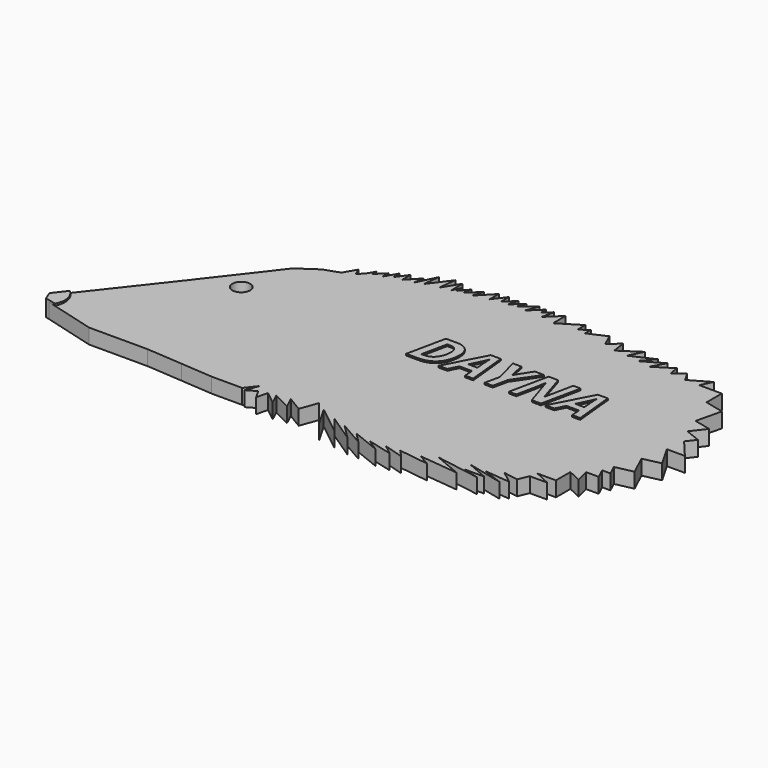
from build123d import *

# Parameters (mm, degrees)
F0_R         = 0.5378033018
F1_DEPTH     = 0.9
F2_TEXT_SIZE = 3.3063238435
F3_DEPTH     = 1
F5_DEPTH     = 1.01


# Not quite as in the source:
# - Text() gives the source's letters only with a copy of the font that has no kerning and outlines rounded to 1/6400 em; it was checked with that copy


with BuildPart() as f1:
    # F0 (on Top) → F1 (new body)
    with BuildSketch(Plane.XY):
        Polygon((-27.0037204027, 5.1291389391), (-31.1524681747, -0.163565157), (-30.9421550483, -0.6564339856), (-27.6378747076, -1.5638275072), (-24.1281446069, -1.5638275072), (-21.9538230449, -1.7179133138), (-20.0191922486, -1.8652107101), (-18.1791530636, -1.8652107101), (-17.6565442234, -1.1985001504), (-17.9531408334, -1.9743070749), (-17.3907472424, -1.6495448565), (-17.0744433999, -2.1972910035), (-16.9113259139, -1.5163020821), (-16.1478312427, -2.1147762757), (-16.4409801364, -1.4782244107), (-15.3690173699, -2.0160753835), (-15.6876724213, -1.3241387205), (-14.780279249, -1.8652107101), (-14.3968500197, -0.8131673094), (-13.0864167586, -2.4542018443), (-13.8115396517, -1.1985001504), (-12.0932376012, -2.5454112329), (-12.8187853843, -1.6203386476), (-11.1681651324, -2.7177287266), (-12.020682916, -1.8652107101), (-10.4970345274, -2.7358673979), (-11.086541228, -2.1372910123), (-9.4268526882, -2.799352631), (-10.1433303207, -2.3368163966), (-8.6197278335, -2.7334264399), (-9.2182578519, -2.2642617114), (-8.0029657111, -2.6270351373), (-8.4055373445, -2.2042002529), (-6.5982462838, -2.448795829), (-7.2912680916, -2.0547248423), (-4.9540190957, -2.299320884), (-6.5574799664, -1.6198880039), (-3.8941039238, -2.0683135372), (-4.8724873923, -1.8101290334), (-3.6630968098, -1.8101290334), (-4.9540190957, -1.2529940577), (-2.7526570484, -1.7829518765), (-3.9892247878, -1.3345261104), (-2.4316561306, -1.484446951), (-3.1603167299, -0.9132778505), (-2.2906428203, -1.0627531447), (-2.0188696217, -0.4376749566), (-0.9725430864, -0.4376749566), (-1.9101604121, 0), (-0.7958906353, 0), (-0.7958906353, 1.0842544725), (0, 0.7173608174), (-0.2115784591, 1.5355834401), (0.54776415, 1.5355834401), (0.2640244784, 2.151703852), (0.7583171951, 2.151703852), (0.4762638127, 2.7641626075), (1.5363685326, 2.9920388722), (0.9654549067, 4.2317369953), (2.0177976039, 4.4688973236), (1.2915831758, 5.7264892384), (2.3786751553, 5.7264892384), (1.4246247635, 6.8606109064), (1.8351287581, 7.3843053542), (0.9124764773, 7.7600274963), (1.5557164371, 8.5806314368), (0.54776415, 8.8206200221), (0.9111003601, 10.3466324508), (-0.2303463552, 10.6184054166), (-0.2303463552, 11.7648066953), (-1.5892117517, 11.7648066953), (-1.2599784476, 12.4465006899), (-2.4404739359, 11.7648066953), (-2.7649223339, 12.3266568407), (-3.3876749221, 11.8695907295), (-3.4910559189, 12.4540766701), (-4.5975148678, 11.7648066953), (-4.1440478526, 12.5810466707), (-5.431894213, 11.8373613805), (-4.7426242381, 12.6173244789), (-6.1211637221, 11.9824707508), (-5.7039740495, 12.816850096), (-6.9011272863, 12.0187476277), (-7.0280982181, 12.8349885345), (-7.6510727601, 12.2644306361), (-7.9894484952, 13.0163757131), (-9.0777678415, 12.5266313553), (-9.0777678415, 12.9800979048), (-9.5856515691, 12.5991860405), (-9.5856515691, 13.1977619603), (-10.8916368335, 12.3996604234), (-10.8916368335, 13.3428713307), (-11.7078768089, 12.5629082322), (-11.5446290001, 13.3065944538), (-12.0162339881, 12.8712663427), (-12.0162339881, 13.2703166455), (-12.7417817712, 12.5629082322), (-12.4334236607, 13.3247328922), (-13.2859414443, 12.6536013559), (-13.0864167586, 13.1614850834), (-13.7394089252, 12.5629082322), (-13.576160185, 13.1433457136), (-14.1747370362, 12.5810466707), (-14.1747370362, 13.1796235219), (-14.7370360792, 12.4359373003), (-14.7370360792, 13.1252072752), (-15.6258307397, 12.2001348063), (-15.4081676155, 12.8531269729), (-16.1325391382, 12.182071805), (-16.0235837102, 12.6784220338), (-16.4715088904, 12.1578592807), (-16.4715088904, 12.5210424885), (-16.7136322707, 12.0125859976), (-16.7136322707, 12.8842266276), (-17.3310432583, 11.8794189766), (-17.2099824995, 12.9447570071), (-18.1179400533, 11.7220394313), (-18.008986488, 12.7026345581), (-18.5900796205, 11.5041295066), (-18.4811241925, 12.1578592807), (-19.1832799464, 11.4193866029), (-19.1832799464, 12.0610101148), (-19.6796301752, 11.3709615543), (-19.6796301752, 11.8431001902), (-20.1033446938, 11.1167337745), (-20.1033446938, 11.5404473618), (-20.6481199712, 10.9956720844), (-20.6481199712, 11.3104311749), (-20.9265593439, 10.8503988013), (-21.2534256279, 10.5114271864), (-21.4350167662, 10.9472479671), (-21.8708366156, 10.208774358), (-22.8030085564, 9.8819099367), (-23.9167697728, 9.1192247346), align=None)
        with Locations((-24.6249865741, 6.1201211065)):
            Circle(F0_R, mode=Mode.SUBTRACT)
    extrude(amount=F1_DEPTH)

    # F2 (on Top) → F3 (join)
    with BuildSketch(Plane.XY):
        with Locations((-14.3002690747, 5.5137877353)):
            Text('DAYNA', F2_TEXT_SIZE, font='Open Sans', font_style=FontStyle.BOLDITALIC, text_align=(TextAlign.LEFT, TextAlign.BOTTOM))
    extrude(amount=F3_DEPTH)

    # F4 (on Top) → F5 (join)
    with BuildSketch(Plane.XY):
        with BuildLine():
            Line((-30.942497775, -0.6605971721), (-30.2765108645, -0.8306366508))
            ThreePointArc((-30.2765108645, -0.8306366508), (-30.1446214755, -0.0546052641), (-30.5351112038, 0.6288691657))
            Line((-30.5351112038, 0.6288691657), (-31.1479624361, -0.1540210942))
            Line((-31.1479624361, -0.1540210942), (-30.942497775, -0.6605971721))
        make_face()
    extrude(amount=F5_DEPTH)


solid = f1.part
